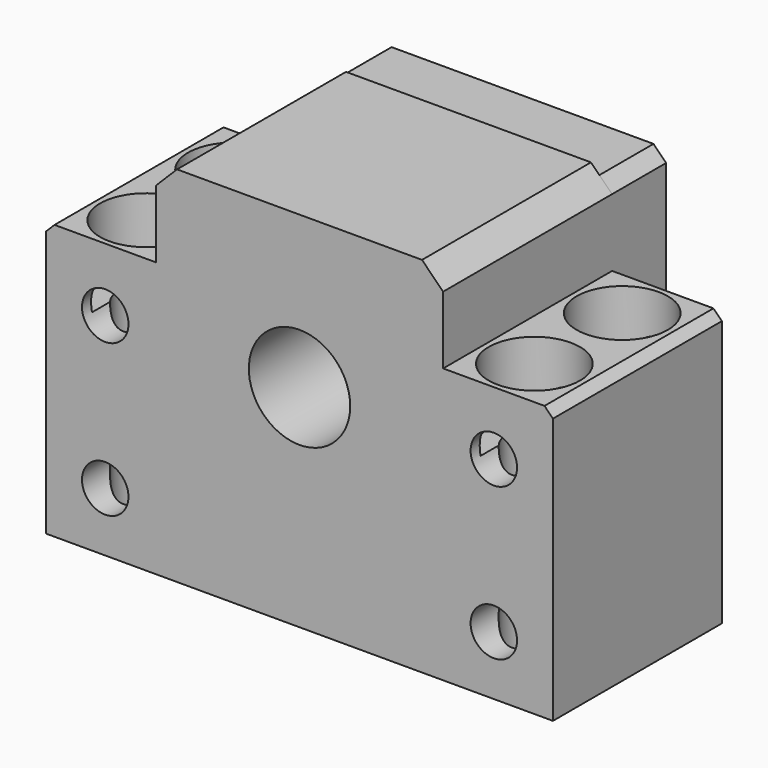
from build123d import *

# Parameters (mm, degrees)
F0_R      = 2.75
F0_R_2    = 6
F1_DEPTH  = 25
F2_SIZE   = 2.5
F3_R      = 5.4
F3_R_2    = 3.3
F4_DEPTH  = 8.5
F5_DEPTH  = 32.501
F6_SIZE   = 1
F7_W      = 34
F7_H      = 34
F7_R      = 6
F8_DEPTH  = 8
F10_SIZE  = 1.49999
F11_R     = 6
F12_DEPTH = 4
F13_SIZE  = 3


# Not quite as in the source:
# - a fillet or chamfer is up to 0.001 mm smaller than in the source, because OpenCascade refuses the exact size
# - a feature of the source that left no trace in its solid (it failed there, or was rolled back) is left out


with BuildPart() as f1:
    # F0 (on Front) → F1 (new body)
    with BuildSketch(Plane.XZ):
        Polygon((-33.4486477077, 0.4262879155), (-37.2326049358, 0.4262879155), (-39.7326049358, 0.4262879155), (-39.7326049358, -32.0737120845), (20.2673950642, -32.0737120845), (20.2673950642, 0.4262879155), (7.2673950642, 0.4262879155), (7.2673950642, 10.9262879155), (-26.7326049358, 10.9262879155), (-26.7326049358, 0.4262879155), align=None)
        with Locations((-32.7326049358, -25.0737120845)):
            Circle(F0_R, mode=Mode.SUBTRACT)
        with Locations((13.2673950642, -25.0737120845)):
            Circle(F0_R, mode=Mode.SUBTRACT)
        with Locations((-32.7326049358, -7.0737120845)):
            Circle(F0_R, mode=Mode.SUBTRACT)
        with Locations((-9.7326049358, -7.0737120845)):
            Circle(F0_R_2, mode=Mode.SUBTRACT)
        with Locations((13.2673950642, -7.0737120845)):
            Circle(F0_R, mode=Mode.SUBTRACT)
    extrude(amount=F1_DEPTH)

    # F2
    f2_edges = [f1.edges().sort_by_distance(p)[0] for p in [
        (-26.732605, -12.5, 10.926288),
        (7.267395, -12.5, 10.926288),
    ]]
    chamfer(f2_edges, length=F2_SIZE)

    # F3 (on face) → F4 (cut)
    with BuildSketch(Plane.XY.offset(0.4262879155)):
        with Locations((13.2673950642, -19)):
            Circle(F3_R)
        with Locations((13.2673950642, -19)):
            Circle(F3_R_2, mode=Mode.SUBTRACT)
        with Locations((13.2673950642, -6)):
            Circle(F3_R)
        with Locations((13.2673950642, -6)):
            Circle(F3_R_2, mode=Mode.SUBTRACT)
        with Locations((-32.7326049358, -6)):
            Circle(F3_R)
        with Locations((-32.7326049358, -6)):
            Circle(F3_R_2, mode=Mode.SUBTRACT)
        with Locations((-32.7326049358, -19)):
            Circle(F3_R)
        with Locations((-32.7326049358, -19)):
            Circle(F3_R_2, mode=Mode.SUBTRACT)
    extrude(amount=-F4_DEPTH, mode=Mode.SUBTRACT)

    # F5 (cut, through all): faces of the model
    f5_faces = [f1.faces().sort_by_distance(p)[0] for p in [
        (13.2673950642, -19, 0.4262879155),
        (13.2673950642, -6, 0.4262879155),
        (-32.7326049358, -6, 0.4262879155),
        (-32.7326049358, -19, 0.4262879155),
    ]]
    extrude(f5_faces, amount=-F5_DEPTH, mode=Mode.SUBTRACT)

    # F6
    f6_edges = [f1.edges().sort_by_distance(p)[0] for p in [
        (20.267395, -12.5, 0.426288),
        (-39.732605, -12.5, 0.426288),
    ]]
    chamfer(f6_edges, length=F6_SIZE)

    # F7 (on face) → F8 (join)
    with BuildSketch(Plane(origin=(0, 0, 0), x_dir=(-1, 0, 0), z_dir=(0, 1, 0))):
        with Locations((9.7326049358, -7.0737120845)):
            Rectangle(F7_W, F7_H)
        with Locations((9.7326049358, -7.0737120845)):
            Circle(F7_R, mode=Mode.SUBTRACT)
    extrude(amount=F8_DEPTH)

    # F10 (size 1.5 in the source; OpenCascade refuses exactly that, so slightly less here)
    f10_edges = [f1.edges().sort_by_distance(p)[0] for p in [
        (-26.732605, 4, 9.926288),
        (7.267395, 4, -24.073712),
        (-26.732605, 4, -24.073712),
        (7.267395, 4, 9.926288),
    ]]
    chamfer(f10_edges, length=F10_SIZE)

    # F11 (on face) → F12 (join)
    with BuildSketch(Plane(origin=(0, 8, 0), x_dir=(-1, 0, 0), z_dir=(0, 1, 0))):
        Polygon((9.7326049358, 4.7399964145), (-1.5811035632, -6.5737120845), (9.7326049358, -17.8874205835), (21.0463134348, -6.5737120845), align=None)
        with Locations((9.7326049358, -7.0737120845)):
            Circle(F11_R, mode=Mode.SUBTRACT)
    extrude(amount=F12_DEPTH)

    # F13
    f13_edges = [f1.edges().sort_by_distance(p)[0] for p in [
        (-9.732605, 10, 4.739996),
        (1.581104, 10, -6.573712),
        (-9.732605, 10, -17.887421),
        (-21.046313, 10, -6.573712),
    ]]
    chamfer(f13_edges, length=F13_SIZE)


solid = f1.part
